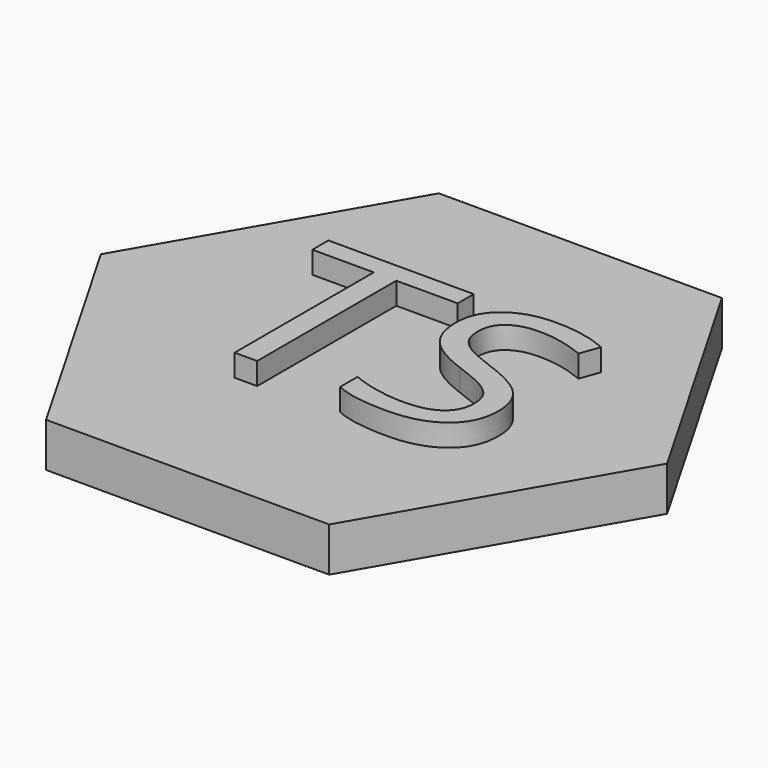
from build123d import *

# Parameters (mm, degrees)
F1_DEPTH     = 10.16
F2_TEXT_SIZE = 62.4090640081
F5_DEPTH     = 15.24


# Not quite as in the source:
# - the program builds the solid bodies; features that only make, move or delete a surface that nothing else refers to are left out
# - Text() gives the source's letters only with a copy of the font that has no kerning and outlines rounded to 1/6400 em; it was checked with that copy


with BuildPart() as f1:
    # F0 (on Top) → F1 (new body)
    with BuildSketch(Plane.XY):
        Polygon((-65.0766651653, 0.0317955258), (-32.5658683158, -56.3421474638), (32.5107968496, -56.3739429897), (65.0766651653, -0.0317955258), (32.5658683158, 56.3421474638), (-32.5107968496, 56.3739429897), align=None)
    extrude(amount=F1_DEPTH)

    # F2 (on Top) → F5 (join)
    with BuildSketch(Plane.XY):
        with Locations((-30.999135226, -22.4672630429)):
            Text('TS', F2_TEXT_SIZE, font='Open Sans', text_align=(TextAlign.LEFT, TextAlign.BOTTOM))
    extrude(amount=F5_DEPTH)


solid = f1.part
